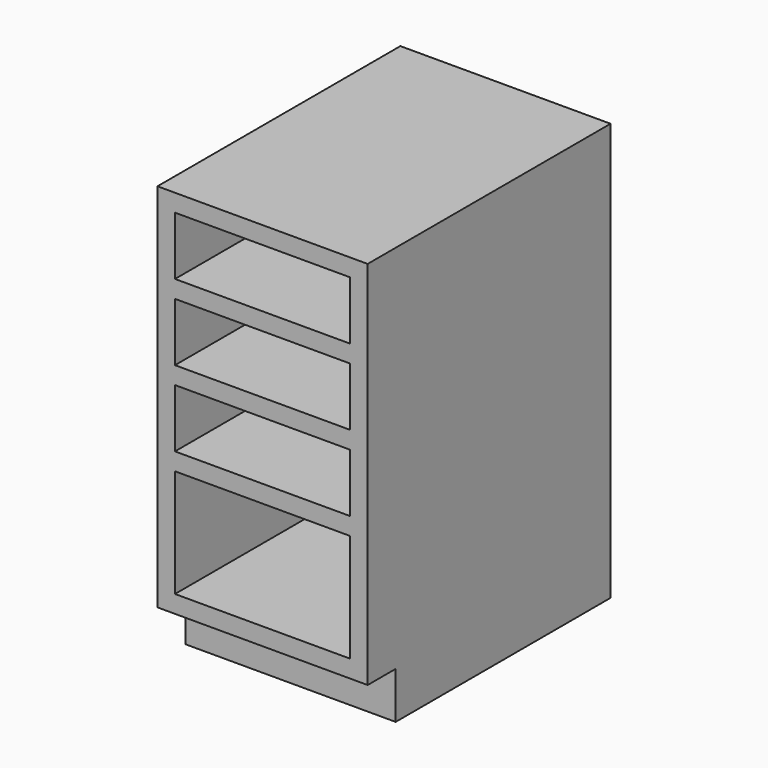
from build123d import *

# Parameters (mm, degrees)
F1_DEPTH = 457.2
F2_W     = 381
F2_H     = 127
F2_H_2   = 234.95
F3_DEPTH = 596.9


# Not quite as in the source:
# - a feature names something its author has since deleted; it is built from what else it names


with BuildPart() as f1:
    # F0 (on Right) → F1 (new body)
    with BuildSketch(Plane.YZ):
        Polygon((-584.2, 0), (0, 0), (0, 908.05), (-660.4, 908.05), (-660.4, 101.6), (-584.2, 101.6), align=None)
    extrude(amount=F1_DEPTH)

    # F2 (on face) → F3 (cut)
    with BuildSketch(Plane.XZ.offset(660.4)):
        with Locations((228.6, 806.45)):
            Rectangle(F2_W, F2_H)
        with Locations((228.6, 641.35)):
            Rectangle(F2_W, F2_H)
        with Locations((228.6, 476.25)):
            Rectangle(F2_W, F2_H)
        with Locations((228.6, 257.175)):
            Rectangle(F2_W, F2_H_2)
    extrude(amount=-F3_DEPTH, mode=Mode.SUBTRACT)


solid = f1.part
